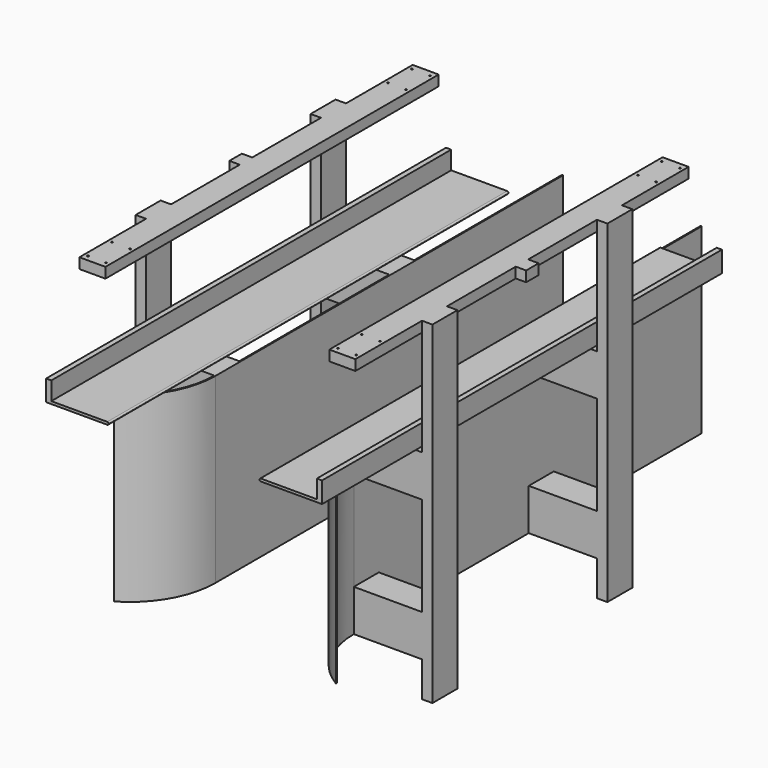
from build123d import *

# Parameters (mm, degrees)
F0_W      = 63.5
F0_H      = 25.4
F1_DEPTH  = 508
F2_W      = 76.2
F2_H      = 812.8
F3_DEPTH  = 25.4
F5_D      = 3.7973
F5_DEPTH  = 15.875
F5_TIP    = 1.1408240143
F7_DEPTH  = 609.6
F8_R      = 3.17499
F9_W      = 76.2
F9_H      = 101.6
F10_DEPTH = 166.37
F12_DEPTH = 444.5
F13_W     = 38.1
F13_H     = 25.4
F14_DEPTH = 25.4


# Not quite as in the source:
# - a fillet or chamfer is up to 0.001 mm smaller than in the source, because OpenCascade refuses the exact size


with BuildPart() as f1:
    # F0 (on Front) → F1 (new body, symmetric)
    with BuildSketch(Plane.XZ):
        Rectangle(F0_W, F0_H)
    extrude(amount=F1_DEPTH, both=True)

    # F2 (on face) → F3 (join)
    with BuildSketch(Plane.YZ.offset(31.75)):
        with Locations((-266.7, -393.7)):
            Rectangle(F2_W, F2_H)
        with Locations((266.7, -393.7)):
            Rectangle(F2_W, F2_H)
    extrude(amount=F3_DEPTH)

    # F5
    with Locations(Plane.XY.offset(12.7)):
        with Locations((22.225, 420.6875), (-22.225, 420.6875), (22.225, 493.7125), (-22.225, 493.7125), (22.225, -420.6875), (-22.225, -420.6875), (-22.225, -493.7125), (22.225, -493.7125)):
            Hole(F5_D / 2, depth=F5_DEPTH)
            with Locations((0, 0, -(F5_DEPTH + F5_TIP / 2))):  # 118° drill point
                Cone(0, F5_D / 2, F5_TIP, mode=Mode.SUBTRACT)

    # F6 (on Front) → F7 (join, symmetric)
    with BuildSketch(Plane.XZ):
        Polygon((-120.65, -257.175), (31.75, -257.175), (31.75, -206.375), (19.05, -206.375), (19.05, -250.825), (-120.65, -250.825), align=None)
    extrude(amount=F7_DEPTH, both=True)

    # F8 (radius 3.175 in the source; OpenCascade refuses exactly that, so slightly less here)
    f8_edges = [f1.edges().sort_by_distance(p)[0] for p in [
        (-120.65, 0, -257.175),
        (-120.65, 0, -250.825),
    ]]
    fillet(f8_edges, radius=F8_R)

    # F9 (on face) → F10 (join)
    with BuildSketch(Plane(origin=(31.75, 0, 0), x_dir=(0, -1, 0), z_dir=(-1, 0, 0))):
        with Locations((-266.7, -320.675)):
            Rectangle(F9_W, F9_H)
        with Locations((266.7, -320.675)):
            Rectangle(F9_W, F9_H)
        with Locations((-266.7, -663.575)):
            Rectangle(F9_W, F9_H)
        with Locations((266.7, -663.575)):
            Rectangle(F9_W, F9_H)
    extrude(amount=F10_DEPTH)

    # F11 (on face) → F12 (join, through all)
    with BuildSketch(Plane.XY.offset(-269.875)):
        with BuildLine():
            ThreePointArc((-33.02, -482.6), (-107.4286784559, -407.1906734034), (-134.62, -304.8))
            Line((-134.62, -304.8), (-134.62, 755.65))
            Line((-134.62, 755.65), (-137.287, 755.65))
            Line((-137.287, 755.65), (-137.287, -304.8))
            ThreePointArc((-137.287, -304.8), (-109.744282916, -408.513875952), (-34.3740153846, -484.8977230769))
            Line((-34.3740153846, -484.8977230769), (-33.02, -482.6))
        make_face()
    extrude(amount=-F12_DEPTH)

    # F13 (on face) → F14 (join, through all)
    with BuildSketch(Plane.YZ.offset(31.75)):
        Rectangle(F13_W, F13_H)
    extrude(amount=F14_DEPTH)


with BuildPart() as f16_1:
    # F16: instance of F1
    add(f1.part.mirror(Plane.YZ.offset(-304.8)))


solid = Compound([f1.part, f16_1.part])
